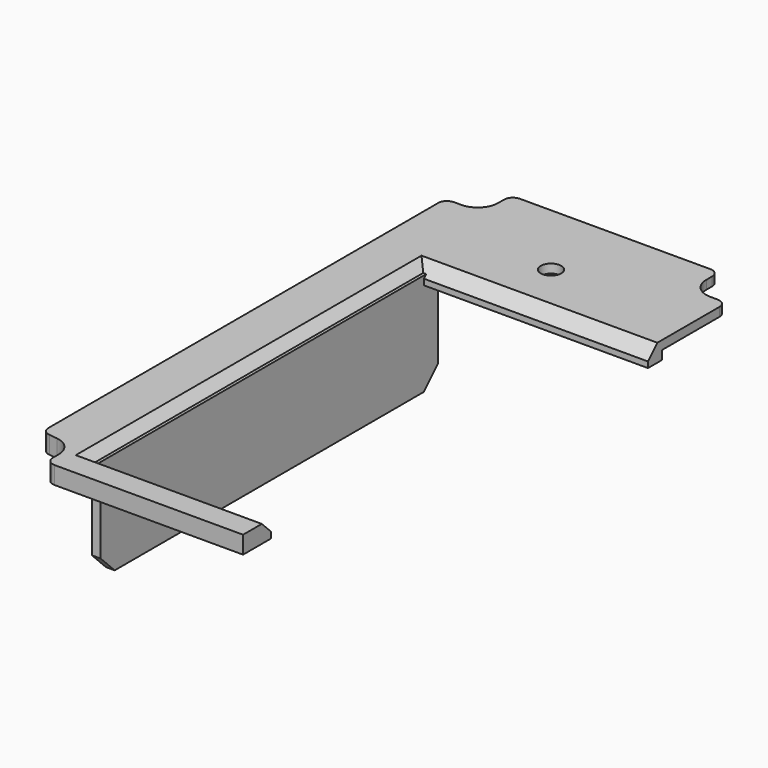
from build123d import *

# Parameters (mm, degrees)
F0_W          = 38.25
F0_H          = 3
F1_DEPTH      = 1.5
F2_DEPTH      = 1.5
F5_DEPTH      = 0.75
F6_R          = 1.5
F7_W          = 1.5
F7_H          = 71.928761142
F8_DEPTH      = 17.5
F10_SIZE      = 3
F13_R         = 1.75
F14_DEPTH     = 25
F15_DEPTH     = 1
F16_T4_DEPTH  = 48.5367319519
F16_T10_DEPTH = 48.5367319519
F16_T15_DEPTH = 80.0367319519
F16_T22_DEPTH = 40.0367319519
F16_T27_DEPTH = 40.0367319519


# Not quite as in the source:
# - a fillet or chamfer that OpenCascade refuses, or shapes differently, is made with other operations: its cross-section is extruded or revolved along the edge and cut away or added


with BuildPart() as f1:
    # F0 (on Top) → F1 (new body)
    with BuildSketch(Plane.XY):
        with BuildLine():
            Line((-14, -42.5426968038), (-23.75, -42.5426968038))
            Line((-23.75, -42.5426968038), (-23.75, -42.9965845553))
            Line((-23.75, -42.9965845553), (-21.0181723213, -43.3122070099))
            ThreePointArc((-21.0181723213, -43.3122070099), (-18.8056300503, -44.4619063855), (-17.919875499, -46.7926982744))
            Line((-17.919875499, -46.7926982744), (-17.9227195281, -49.5426968038))
            Line((-17.9227195281, -49.5426968038), (15.75, -49.5426968038))
            Line((15.75, -49.5426968038), (15.75, -42.5426968038))
            Line((15.75, -42.5426968038), (-14, -42.5426968038))
        make_face()
        with BuildLine():
            Line((18, 49.2073031962), (-17.5, 49.2073031962))
            Line((-17.5, 49.2073031962), (-17.5, 46.4573031962))
            ThreePointArc((-17.5, 46.4573031962), (-18.5251262658, 43.982429462), (-21, 42.9573031962))
            Line((-21, 42.9573031962), (-23.75, 42.9573031962))
            Line((-23.75, 42.9573031962), (-23.75, -42.5426968038))
            Line((-23.75, -42.5426968038), (-14, -42.5426968038))
            Line((-14, -42.5426968038), (-14, 26.2073031962))
            Line((-14, 26.2073031962), (-14, 29.2073031962))
            Line((-14, 29.2073031962), (24.25, 29.2073031962))
            Line((24.25, 29.2073031962), (24.25, 42.9570424259))
            Line((24.25, 42.9570424259), (21.4996681305, 42.9573032119))
            ThreePointArc((21.4996681305, 42.9573032119), (19.0250089351, 43.9825467984), (18, 46.4573031962))
            Line((18, 46.4573031962), (18, 49.2073031962))
        make_face()
        with Locations((5.125, 27.7073031962)):
            Rectangle(F0_W, F0_H)
    extrude(amount=F1_DEPTH)

    # F0 (on Top) → F2 (join)
    with BuildSketch(Plane.XY):
        with BuildLine():
            Line((-14, -42.5426968038), (-23.75, -42.5426968038))
            Line((-23.75, -42.5426968038), (-23.75, -42.9965845553))
            Line((-23.75, -42.9965845553), (-21.0181723213, -43.3122070099))
            ThreePointArc((-21.0181723213, -43.3122070099), (-18.8056300503, -44.4619063855), (-17.919875499, -46.7926982744))
            Line((-17.919875499, -46.7926982744), (-17.9227195281, -49.5426968038))
            Line((-17.9227195281, -49.5426968038), (15.75, -49.5426968038))
            Line((15.75, -49.5426968038), (15.75, -42.5426968038))
            Line((15.75, -42.5426968038), (-14, -42.5426968038))
        make_face()
        with Locations((5.125, 27.7073031962)):
            Rectangle(F0_W, F0_H)
    extrude(amount=-F2_DEPTH)

    # F3: union 

    # F4 (on face) → F5 (cut)
    with BuildSketch(Plane.XY):
        Polygon((-19.8072306812, 41.2358827889), (-27.7905139636, 41.2358827889), (-27.9461211857, -15.0937307626), (-19.8072306812, -15.0937307626), align=None)
    extrude(amount=F5_DEPTH, mode=Mode.SUBTRACT)

    # F6
    f6_edges = [f1.edges().sort_by_distance(p)[0] for p in [
        (-17.5, 49.207303, 0.75),
        (-23.75, 42.957303, 0.75),
        (18, 49.207303, 0.75),
        (24.25, 42.957042, 0.75),
        (-23.75, -42.996585, 0),
        (-17.92272, -49.542697, 0),
    ]]
    fillet(f6_edges, radius=F6_R)

    # F7 (on Top) → F8 (join)
    with BuildSketch(Plane.XY):
        with Locations((-14.7299332246, -6.7935563562)):
            Rectangle(F7_W, F7_H)
    extrude(amount=-F8_DEPTH)

    # F9: union 

    # F10
    f10_edges = [f1.edges().sort_by_distance(p)[0] for p in [
        (-14.729933, -42.757937, -17.5),
        (-14.729933, 29.170824, -17.5),
    ]]
    chamfer(f10_edges, length=F10_SIZE)


with BuildPart() as f11_1:
    # F11: copy of F1
    add(f1.part)


with BuildPart() as f1_1:
    add(f1.part)

    # F13 (on face) → F14 (cut)
    with BuildSketch(Plane.XY.offset(1.5)):
        with Locations((5.438e-07, 35.8340851963)):
            Circle(F13_R)
    extrude(amount=-F14_DEPTH, mode=Mode.SUBTRACT)

    # F15 (cut): a face of the model
    f15_faces = [f1_1.faces().sort_by_distance(p)[0] for p in [
        (0.8800150014, -42.5426968038, 0.0002530279),
    ]]
    extrude(f15_faces, amount=-F15_DEPTH, mode=Mode.SUBTRACT)

    # F16: chamfer of 2 on 3 edges, made by hand


with BuildPart() as f16_tool2:
    # F16_s3 → F16_t4 (new body)
    with BuildSketch(Plane.YZ.offset(-19.1433659759)):
        Polygon((28.2073031962, 1.5), (26.2073031962, -0.5), (26.2073031962, 1.5), align=None)
    extrude(amount=F16_T4_DEPTH)

    split(bisect_by=Plane.XY, keep=Keep.TOP)

    split(bisect_by=Plane(origin=(-7.25, 0, -7.25), x_dir=(0, 1, 0), z_dir=(0.7071067812, 0, 0.7071067812)), keep=Keep.TOP)


with BuildPart() as f1_2:
    add(f1_1.part)

    # F16_t1: cut F16_tool2
    add(f16_tool2.part, mode=Mode.SUBTRACT)


with BuildPart() as f16_tool8:
    # F16_s9 → F16_t10 (new body)
    with BuildSketch(Plane.YZ.offset(-19.1433659759)):
        Polygon((28.2073031962, 1.5), (26.2073031962, -0.5), (26.2073031962, 1.5), align=None)
    extrude(amount=F16_T10_DEPTH)

    split(bisect_by=Plane.YZ.offset(-13.9799332246), keep=Keep.TOP)


with BuildPart() as f1_3:
    add(f1_2.part)

    # F16_t7: cut F16_tool8
    add(f16_tool8.part, mode=Mode.SUBTRACT)


with BuildPart() as f16_tool13:
    # F16_s14 → F16_t15 (new body)
    with BuildSketch(Plane.XZ.offset(48.6860627797)):
        Polygon((-14, -0.5), (-16, 1.5), (-14, 1.5), align=None)
    extrude(amount=-F16_T15_DEPTH)

    split(bisect_by=Plane.XY, keep=Keep.TOP)

    split(bisect_by=Plane(origin=(0, 13.3536515981, -13.3536515981), x_dir=(1, 0, 0), z_dir=(0, -0.7071067812, 0.7071067812)), keep=Keep.TOP)

    split(bisect_by=Plane(origin=(0, -22.0213484019, -22.0213484019), x_dir=(1, 0, 0), z_dir=(0, 0.7071067812, 0.7071067812)), keep=Keep.TOP)


with BuildPart() as f1_4:
    add(f1_3.part)

    # F16_t12: cut F16_tool13
    add(f16_tool13.part, mode=Mode.SUBTRACT)


with BuildPart() as f16_tool20:
    # F16_s21 → F16_t22 (new body)
    with BuildSketch(Plane.YZ.offset(20.8933659759)):
        Polygon((-43.5426968038, -0.5), (-45.5426968038, 1.5), (-43.5426968038, 1.5), align=None)
    extrude(amount=-F16_T22_DEPTH)

    split(bisect_by=Plane.YZ.offset(-13.9799332246), keep=Keep.TOP)


with BuildPart() as f1_5:
    add(f1_4.part)

    # F16_t19: cut F16_tool20
    add(f16_tool20.part, mode=Mode.SUBTRACT)


with BuildPart() as f16_tool25:
    # F16_s26 → F16_t27 (new body)
    with BuildSketch(Plane.YZ.offset(20.8933659759)):
        Polygon((-43.5426968038, -0.5), (-45.5426968038, 1.5), (-43.5426968038, 1.5), align=None)
    extrude(amount=-F16_T27_DEPTH)

    split(bisect_by=Plane.XY, keep=Keep.TOP)

    split(bisect_by=Plane(origin=(-7.25, 0, -7.25), x_dir=(0, 1, 0), z_dir=(0.7071067812, 0, 0.7071067812)), keep=Keep.TOP)


with BuildPart() as f1_6:
    add(f1_5.part)

    # F16_t24: cut F16_tool25
    add(f16_tool25.part, mode=Mode.SUBTRACT)


solid = f1_6.part
